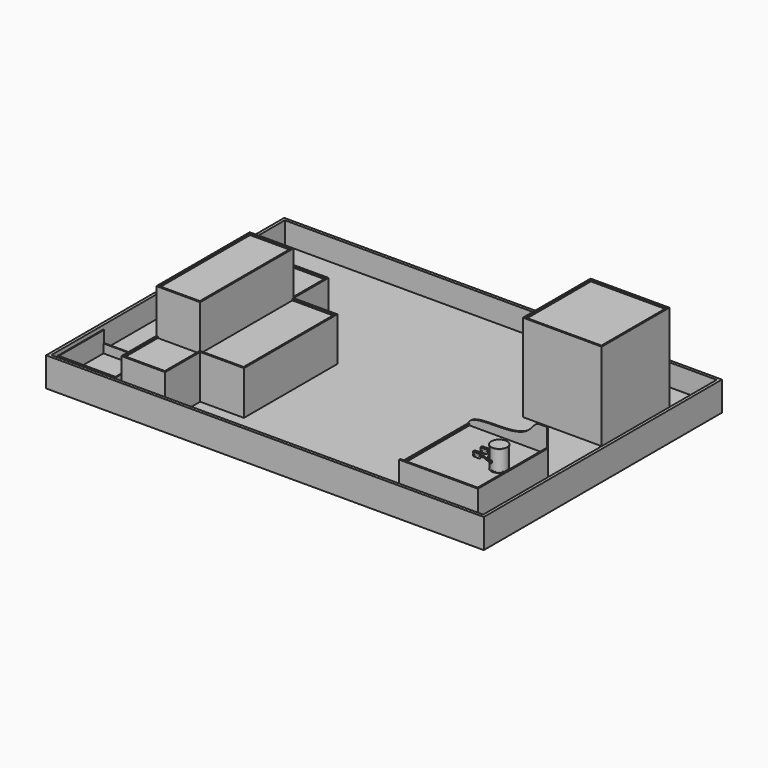
from build123d import *

# Parameters (mm, degrees)
F0_R      = 27.2
F1_DEPTH  = 2.83
F2_R      = 26.4
F3_DEPTH  = 67.36
F4_R      = 27.2
F5_DEPTH  = 2.83
F9_W      = 270
F9_H      = 300
F10_DEPTH = 72
F12_DEPTH = 15
F14_DEPTH = 5
F15_W     = 5
F15_H     = 290
F16_DEPTH = 5
F17_W     = 1500
F17_H     = 1020
F18_DEPTH = 25
F19_W     = 270
F19_H     = 290
F20_DEPTH = 300
F21_W     = 260
F21_H     = 280
F22_DEPTH = 5
F23_W     = 1500
F23_H     = 1020
F23_W_2   = 1480
F23_H_2   = 1000
F24_DEPTH = 75
F26_DEPTH = 150
F27_W     = 150
F27_H     = 400
F28_DEPTH = 150
F29_W     = 140
F29_H     = 390
F30_DEPTH = 5
F31_W     = 140
F31_H     = 145
F31_W_2   = 145
F31_H_2   = 390
F32_DEPTH = 5
F33_R     = 3
F34_DEPTH = 4
F35_R     = 3.99999
F35_2_R   = 3.99999
F36_R     = 3
F37_DEPTH = 8
F38_R     = 3
F39_DEPTH = 8
F40_R     = 3
F40_R_2   = 2.5
F41_DEPTH = 3
F42_R     = 3
F42_R_2   = 2.5
F43_DEPTH = 3
F45_DEPTH = 270.001
F46_W     = 200
F46_H     = 200
F46_W_2   = 194
F46_H_2   = 191
F47_DEPTH = 30
F49_DEPTH = 40
F50_R     = 2.5903397147
F50_R_2   = 2.8335127801
F50_R_3   = 2.8175430484
F50_R_4   = 2.711905074
F51_DEPTH = 6


# Not quite as in the source:
# - a fillet or chamfer is up to 0.001 mm smaller than in the source, because OpenCascade refuses the exact size
# - a feature names something its author has since deleted; it is built from what else it names


with BuildPart() as f1:
    # F0 (on Top) → F1 (new body)
    with BuildSketch(Plane.XY):
        Circle(F0_R)
    extrude(amount=F1_DEPTH)

    # F2 (on face) → F3 (join)
    with BuildSketch(Plane.XY.offset(2.83)):
        Circle(F2_R)
    extrude(amount=F3_DEPTH)

    # F4 (on face) → F5 (join)
    with BuildSketch(Plane.XY.offset(70.19)):
        Circle(F4_R)
    extrude(amount=F5_DEPTH)


with BuildPart() as f10:
    # F9 (on Top) → F10 (new body)
    with BuildSketch(Plane.XY):
        with Locations((-87.8, 0)):
            Rectangle(F9_W, F9_H)
    extrude(amount=-F10_DEPTH)

    # F11 (on face) → F12 (join)
    with BuildSketch(Plane.XY):
        Polygon((-222.8, -145), (-222.8, -150), (47.2, -150), (47.2, 150), (42.2, 150), (42.2, -145), align=None)
    extrude(amount=F12_DEPTH)

    # F13 (on face) → F14 (join)
    with BuildSketch(Plane(origin=(0, 150, 0), x_dir=(-1, 0, 0), z_dir=(0, 1, 0))):
        with BuildLine():
            Line((-21.3134280931, 81.3575685024), (-47.2, 81.3575685024))
            Line((-47.2, 81.3575685024), (-47.2, -72))
            Line((-47.2, -72), (222.8, -72))
            Line((222.8, -72), (222.8, 0))
            add(Edge.make_bspline(
                [(-21.3134280931, 81.3575685024), (-6.3059147253, 81.3822787863), (12.9585432644, 38.1268753575), (103.6097013063, 23.6068887567), (223.0224295336, 30.7718731823), (222.8, 0)],
                knots=[0, 0, 0, 0, 0.2487100673, 0.6151112321, 1, 1, 1, 1], degree=3))
        make_face()
    extrude(amount=-F14_DEPTH)

    # F15 (on face) → F16 (join)
    with BuildSketch(Plane.XY):
        with Locations((-220.3, 0)):
            Rectangle(F15_W, F15_H)
    extrude(amount=F16_DEPTH)

    # F17 (on face) → F18 (join)
    with BuildSketch(Plane(origin=(0, 0, -72), x_dir=(1, 0, 0), z_dir=(0, 0, -1))):
        with Locations((-602.8, -260)):
            Rectangle(F17_W, F17_H)
    extrude(amount=F18_DEPTH)

    # F19 (on face) → F20 (join)
    with BuildSketch(Plane.XY.offset(-72)):
        with Locations((-87.8, 525)):
            Rectangle(F19_W, F19_H)
    extrude(amount=F20_DEPTH)

    # F21 (on face) → F22 (cut)
    with BuildSketch(Plane.XY.offset(228)):
        with Locations((-87.8, 525)):
            Rectangle(F21_W, F21_H)
    extrude(amount=-F22_DEPTH, mode=Mode.SUBTRACT)

    # F23 (on face) → F24 (join)
    with BuildSketch(Plane.XY.offset(-72)):
        with Locations((-602.8, 260)):
            Rectangle(F23_W, F23_H)
        with Locations((-602.8, 260)):
            Rectangle(F23_W_2, F23_H_2, mode=Mode.SUBTRACT)
    extrude(amount=F24_DEPTH)

    # F25 (on face) → F26 (join)
    with BuildSketch(Plane.XY.offset(-72)):
        Polygon((-952.8, 460), (-1102.8, 460), (-1102.8, -240), (-952.8, -240), (-952.8, -90), (-802.8, -90), (-802.8, 310), (-952.8, 310), align=None)
    extrude(amount=F26_DEPTH)

    # F27 (on face) → F28 (join)
    with BuildSketch(Plane.XY.offset(78)):
        with Locations((-1027.8, 110)):
            Rectangle(F27_W, F27_H)
    extrude(amount=F28_DEPTH)

    # F29 (on face) → F30 (cut)
    with BuildSketch(Plane.XY.offset(228)):
        with Locations((-1027.8, 110)):
            Rectangle(F29_W, F29_H)
    extrude(amount=-F30_DEPTH, mode=Mode.SUBTRACT)

    # F31 (on face) → F32 (cut)
    with BuildSketch(Plane.XY.offset(78)):
        with Locations((-1027.8, 382.5)):
            Rectangle(F31_W, F31_H)
        with Locations((-880.3, 110)):
            Rectangle(F31_W_2, F31_H_2)
        with Locations((-1027.8, -162.5)):
            Rectangle(F31_W, F31_H)
    extrude(amount=-F32_DEPTH, mode=Mode.SUBTRACT)

    # F46 (on face) → F47 (join)
    with BuildSketch(Plane.XY.offset(-72)):
        with Locations((-1232.8, -130)):
            Rectangle(F46_W, F46_H)
        with Locations((-1232.8, -128.5)):
            Rectangle(F46_W_2, F46_H_2, mode=Mode.SUBTRACT)
    extrude(amount=F47_DEPTH)

    # F48 (on face) → F49 (join)
    with BuildSketch(Plane.XY.offset(-42)):
        Polygon((-1329.8, -30), (-1332.8, -30), (-1332.8, -230), (-1329.8, -230), (-1135.8, -230), (-1132.8, -230), (-1132.8, -30), (-1135.8, -30), (-1135.8, -224), (-1329.8, -224), align=None)
    extrude(amount=F49_DEPTH)


with BuildPart() as f34:
    # F33 (on offset) → F34 (new body, symmetric)
    with BuildSketch(Plane.XY.offset(25)):
        with BuildLine():
            Line((-55, -12), (-74.5, -12))
            Line((-74.5, -12), (-74.5, -13))
            Line((-74.5, -13), (-65.6457513111, -13))
            ThreePointArc((-65.6457513111, -13), (-67, -16), (-65.6457513111, -19))
            Line((-65.6457513111, -19), (-74.5, -19))
            Line((-74.5, -19), (-74.5, -20))
            Line((-74.5, -20), (-55, -20))
            ThreePointArc((-55, -20), (-51, -16), (-55, -12))
        make_face()
        with Locations((-63, -16)):
            Circle(F33_R, mode=Mode.SUBTRACT)
        with Locations((-55, -16)):
            Circle(F33_R, mode=Mode.SUBTRACT)
    extrude(amount=F34_DEPTH, both=True)

    # F35 (radius 4 in the source; OpenCascade refuses exactly that, so slightly less here)
    f35_edges = [f34.edges().sort_by_distance(p)[0] for p in [
        (-74.5, -19.5, 29),
        (-74.5, -12.5, 29),
        (-74.5, -19.5, 21),
        (-74.5, -12.5, 21),
    ]]
    fillet(f35_edges, radius=F35_R)

    # F36 (on face) → F37 (join, through all)
    with BuildSketch(Plane.XZ.offset(20)):
        with Locations((-70.5, 25)):
            Circle(F36_R)
    extrude(amount=-F37_DEPTH)

    # F42 (on offset) → F43 (join, symmetric)
    with BuildSketch(Plane.XY.offset(25)):
        with Locations((-63, -16)):
            Circle(F42_R)
        with Locations((-63, -16)):
            Circle(F42_R_2, mode=Mode.SUBTRACT)
        with Locations((-55, -16)):
            Circle(F42_R)
        with Locations((-55, -16)):
            Circle(F42_R_2, mode=Mode.SUBTRACT)
    extrude(amount=F43_DEPTH, both=True)


with BuildPart() as f34b:
    # F33 (on offset) → F34, piece 2 (new body, symmetric)
    with BuildSketch(Plane.XY.offset(25)):
        with BuildLine():
            Line((-74.5, 13), (-74.5, 12))
            Line((-74.5, 12), (-55, 12))
            ThreePointArc((-55, 12), (-51, 16), (-55, 20))
            Line((-55, 20), (-74.5, 20))
            Line((-74.5, 20), (-74.5, 19))
            Line((-74.5, 19), (-65.6457513111, 19))
            ThreePointArc((-65.6457513111, 19), (-67, 16), (-65.6457513111, 13))
            Line((-65.6457513111, 13), (-74.5, 13))
        make_face()
        with Locations((-63, 16)):
            Circle(F33_R, mode=Mode.SUBTRACT)
        with Locations((-55, 16)):
            Circle(F33_R, mode=Mode.SUBTRACT)
    extrude(amount=F34_DEPTH, both=True)

    # F35#2 (radius 4 in the source; OpenCascade refuses exactly that, so slightly less here)
    f35_2_edges = [f34b.edges().sort_by_distance(p)[0] for p in [
        (-74.5, 12.5, 29),
        (-74.5, 19.5, 29),
        (-74.5, 19.5, 21),
        (-74.5, 12.5, 21),
    ]]
    fillet(f35_2_edges, radius=F35_2_R)

    # F38 (on face) → F39 (join, through all)
    with BuildSketch(Plane(origin=(0, 20, 0), x_dir=(-1, 0, 0), z_dir=(0, 1, 0))):
        with Locations((70.5, 25)):
            Circle(F38_R)
    extrude(amount=-F39_DEPTH)

    # F40 (on offset) → F41 (join, symmetric)
    with BuildSketch(Plane.XY.offset(25)):
        with Locations((-55, 16)):
            Circle(F40_R)
        with Locations((-55, 16)):
            Circle(F40_R_2, mode=Mode.SUBTRACT)
        with Locations((-63, 16)):
            Circle(F40_R)
        with Locations((-63, 16)):
            Circle(F40_R_2, mode=Mode.SUBTRACT)
    extrude(amount=F41_DEPTH, both=True)


with BuildPart() as f45_tool:
    # F44 (on face) → F45 (new body, through all)
    with BuildSketch(Plane(origin=(0, 20, 0), x_dir=(-1, 0, 0), z_dir=(0, 1, 0))):
        with BuildLine():
            Line((71.5, 26), (71.5, 27.2912878475))
            ThreePointArc((71.5, 27.2912878475), (70.5, 27.5), (69.5, 27.2912878475))
            Line((69.5, 27.2912878475), (69.5, 26))
            Line((69.5, 26), (68.2087121525, 26))
            ThreePointArc((68.2087121525, 26), (68, 25), (68.2087121525, 24))
            Line((68.2087121525, 24), (69.5, 24))
            Line((69.5, 24), (69.5, 22.7087121525))
            ThreePointArc((69.5, 22.7087121525), (70.5, 22.5), (71.5, 22.7087121525))
            Line((71.5, 22.7087121525), (71.5, 24))
            Line((71.5, 24), (72.7912878475, 24))
            ThreePointArc((72.7912878475, 24), (73, 25), (72.7912878475, 26))
            Line((72.7912878475, 26), (71.5, 26))
        make_face()
    extrude(amount=-F45_DEPTH)


with BuildPart() as f34_1:
    add(f34.part)

    # F45: cut by f45_tool
    add(f45_tool.part, mode=Mode.SUBTRACT)


with BuildPart() as f34b_1:
    add(f34b.part)

    # F45: cut by f45_tool
    add(f45_tool.part, mode=Mode.SUBTRACT)


with BuildPart() as f51:
    # F50 (on face) → F51 (new body)
    with BuildSketch(Plane.XY.offset(29)):
        with BuildLine():
            Line((-35.5209745467, 20), (-70.8834237456, 20))
            ThreePointArc((-70.8834237456, 20), (-73.7118508704, 18.8284271247), (-74.8834237456, 16))
            Line((-74.8834237456, 16), (-74.8834237456, 15.3105559722))
            ThreePointArc((-74.8834237456, 15.3105559722), (-73.7118508704, 12.4821288474), (-70.8834237456, 11.3105559722))
            Line((-70.8834237456, 11.3105559722), (-39.5209745467, 11.3105559722))
            ThreePointArc((-39.5209745467, 11.3105559722), (-36.6925474219, 10.1389830969), (-35.5209745467, 7.3105559722))
            Line((-35.5209745467, 7.3105559722), (-35.5209745467, -7.1426720396))
            ThreePointArc((-35.5209745467, -7.1426720396), (-36.6925474219, -9.9710991643), (-39.5209745467, -11.1426720396))
            Line((-39.5209745467, -11.1426720396), (-70.8834237456, -11.1426720396))
            ThreePointArc((-70.8834237456, -11.1426720396), (-73.7118508704, -12.3142449148), (-74.8834237456, -15.1426720396))
            Line((-74.8834237456, -15.1426720396), (-74.8834237456, -16.5674823374))
            ThreePointArc((-74.8834237456, -16.5674823374), (-73.7118508704, -19.3959094621), (-70.8834237456, -20.5674823374))
            Line((-70.8834237456, -20.5674823374), (-35.5209745467, -20.5674823374))
            Line((-35.5209745467, -20.5674823374), (-0.5937266396, -36.3679043949))
            Line((-0.5937266396, -36.3679043949), (-0.5937266396, -29.9922954291))
            ThreePointArc((-0.5937266396, -29.9922954291), (-29.4402401953, -0.8606840494), (-1.7025308916, 29.3285790831))
            Line((-1.7025308916, 29.3285790831), (-1.7025308916, 37.090189755))
            Line((-1.7025308916, 37.090189755), (-35.5209745467, 20))
        make_face()
        with Locations((-63, -16)):
            Circle(F50_R, mode=Mode.SUBTRACT)
        with Locations((-55.0190731883, -16.1279235035)):
            Circle(F50_R_2, mode=Mode.SUBTRACT)
        with Locations((-63, 16)):
            Circle(F50_R_3, mode=Mode.SUBTRACT)
        with Locations((-55, 16)):
            Circle(F50_R_4, mode=Mode.SUBTRACT)
    extrude(amount=F51_DEPTH)


solid = Compound([f1.part, f10.part, f34_1.part, f34b_1.part, f51.part])
